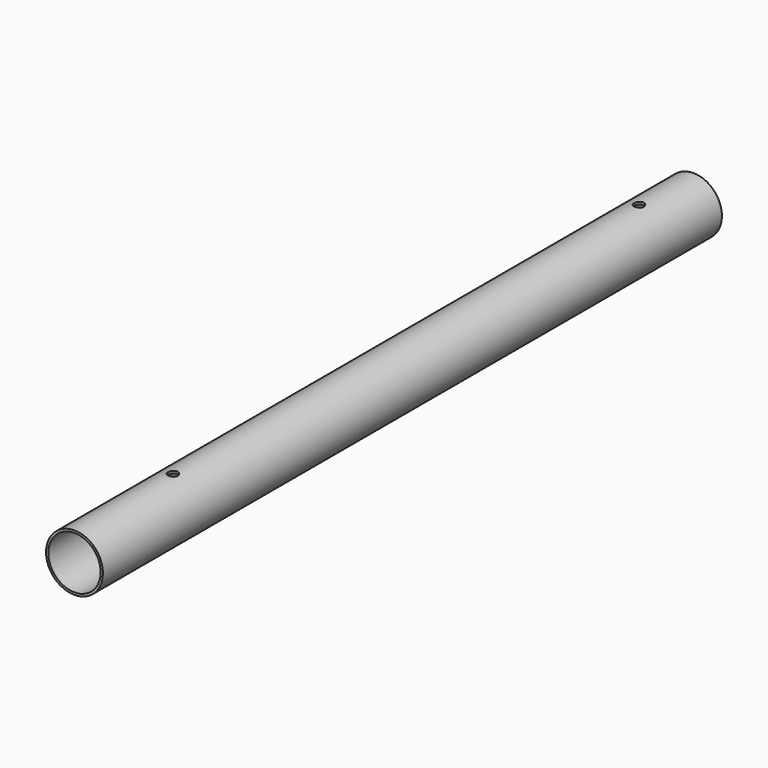
from build123d import *

# Parameters (mm, degrees)
F0_R     = 12.5
F0_R_2   = 11.5
F1_DEPTH = 340
F3_D     = 4.4
F3_DEPTH = 12.501


# Not quite as in the source:
# - a feature names something its author has since deleted; it is built from what else it names


with BuildPart() as f1:
    # F0 (on Front) → F1 (new body)
    with BuildSketch(Plane.XZ):
        Circle(F0_R)
        Circle(F0_R_2, mode=Mode.SUBTRACT)
    extrude(amount=F1_DEPTH)

    # F3 (through all, one way)
    with BuildSketch(Plane(origin=(0, 0, 0), x_dir=(1, 0, 0), z_dir=(0, 0, -1))):
        with Locations((0, 30), (0, 286)):
            Circle(F3_D / 2)
    extrude(amount=-F3_DEPTH, mode=Mode.SUBTRACT)


solid = f1.part
